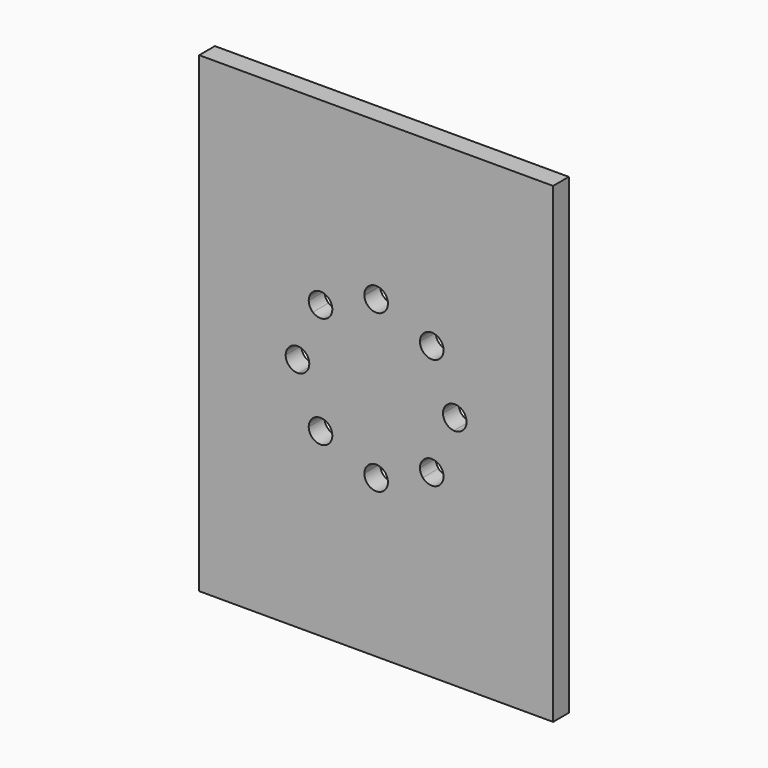
from build123d import *

# Parameters (mm, degrees)
F1_DEPTH = 5
F3_DEPTH = 5
F4_R     = 30
F5_DEPTH = 5
F6_DEPTH = 10


# Not quite as in the source:
# - a feature names something its author has since deleted; it is built from what else it names


with BuildPart() as f1:
    # F0 (on Front) → F1 (new body)
    with BuildSketch(Plane.XZ):
        Polygon((45, 60), (-45, 60), (-45, 0), (-45, -60), (0, -60), (45, -60), align=None)
    extrude(amount=F1_DEPTH)


with BuildPart() as f3:
    # F2 (on face) → F3 (new body)
    with BuildSketch(Plane(origin=(0, 0, 0), x_dir=(-1, 0, 0), z_dir=(0, 1, 0))):
        with BuildLine():
            Line((-40, -45), (-18, -55))
            Line((-18, -55), (18, -55))
            Line((18, -55), (18, -45))
            ThreePointArc((18, -45), (23.4818815859, -37.7525512861), (32.1421356237, -35))
            Line((32.1421356237, -35), (40, -35))
            Line((40, -35), (40, 35))
            Line((40, 35), (33, 35))
            ThreePointArc((33, 35), (22.3933982822, 39.3933982822), (18, 50))
            Line((18, 50), (18, 55))
            Line((18, 55), (-25, 55))
            ThreePointArc((-25, 55), (-35.6066017178, 50.6066017178), (-40, 40))
            Line((-40, 40), (-40, -45))
        make_face()
    extrude(amount=F3_DEPTH)

    # F4 (on face) → F5 (cut)
    with BuildSketch(Plane(origin=(0, 5, 0), x_dir=(-1, 0, 0), z_dir=(0, 1, 0))):
        Circle(F4_R)
        with BuildLine():
            ThreePointArc((16.1001741522, 11.8652598905), (18.4781684496, 7.6522735674), (19.775, 2.9915506013))
            ThreePointArc((19.775, 2.9915506013), (22.0402205763, 2.1994317448), (23, 0))
            ThreePointArc((23, 0), (22.0402205763, -2.1994317448), (19.775, -2.9915506013))
            ThreePointArc((19.775, -2.9915506013), (18.4781684496, -7.6522735674), (16.1001741522, -11.8652598905))
            ThreePointArc((16.1001741522, -11.8652598905), (16.8707805694, -12.8885427857), (17.144270925, -14.14))
            ThreePointArc((17.144270925, -14.14), (15.187715229, -16.9526898131), (11.870121602, -16.0965901095))
            ThreePointArc((11.870121602, -16.0965901095), (7.6550636836, -18.4770127456), (2.9915506013, -19.775))
            ThreePointArc((2.9915506013, -19.775), (2.9978869061, -19.8874207031), (3, -20))
            ThreePointArc((3, -20), (-0.1125792969, -22.9978869061), (-2.9915506013, -19.775))
            ThreePointArc((-2.9915506013, -19.775), (-7.6550636836, -18.4770127456), (-11.870121602, -16.0965901095))
            ThreePointArc((-11.870121602, -16.0965901095), (-16.2659115638, -16.261), (-16.1001741522, -11.8652598905))
            ThreePointArc((-16.1001741522, -11.8652598905), (-18.4781684496, -7.6522735674), (-19.775, -2.9915506013))
            ThreePointArc((-19.775, -2.9915506013), (-23, 0), (-19.775, 2.9915506013))
            ThreePointArc((-19.775, 2.9915506013), (-18.4781684496, 7.6522735674), (-16.1001741522, 11.8652598905))
            ThreePointArc((-16.1001741522, 11.8652598905), (-16.2659115638, 16.261), (-11.870121602, 16.0965901095))
            ThreePointArc((-11.870121602, 16.0965901095), (-7.6550636836, 18.4770127456), (-2.9915506013, 19.775))
            ThreePointArc((-2.9915506013, 19.775), (-0.1125792969, 22.9978869061), (3, 20))
            ThreePointArc((3, 20), (2.9978869061, 19.8874207031), (2.9915506013, 19.775))
            ThreePointArc((2.9915506013, 19.775), (7.6550636836, 18.4770127456), (11.870121602, 16.0965901095))
            ThreePointArc((11.870121602, 16.0965901095), (15.187715229, 16.9526898131), (17.144270925, 14.14))
            ThreePointArc((17.144270925, 14.14), (16.8707805694, 12.8885427857), (16.1001741522, 11.8652598905))
        make_face(mode=Mode.SUBTRACT)
        with BuildLine():
            ThreePointArc((19.775, -2.9915506013), (17, 0), (19.775, 2.9915506013))
            ThreePointArc((19.775, 2.9915506013), (18.4781684496, 7.6522735674), (16.1001741522, 11.8652598905))
            ThreePointArc((16.1001741522, 11.8652598905), (12.0226302863, 12.019), (11.870121602, 16.0965901095))
            ThreePointArc((11.870121602, 16.0965901095), (7.6550636836, 18.4770127456), (2.9915506013, 19.775))
            ThreePointArc((2.9915506013, 19.775), (0, 17), (-2.9915506013, 19.775))
            ThreePointArc((-2.9915506013, 19.775), (-7.6550636836, 18.4770127456), (-11.870121602, 16.0965901095))
            ThreePointArc((-11.870121602, 16.0965901095), (-11.3315811119, 15.183444304), (-11.144270925, 14.14))
            ThreePointArc((-11.144270925, 14.14), (-12.8928137107, 11.4134903556), (-16.1001741522, 11.8652598905))
            ThreePointArc((-16.1001741522, 11.8652598905), (-18.4781684496, 7.6522735674), (-19.775, 2.9915506013))
            ThreePointArc((-19.775, 2.9915506013), (-17.8005682552, 2.0402205763), (-17, 0))
            ThreePointArc((-17, 0), (-17.8005682552, -2.0402205763), (-19.775, -2.9915506013))
            ThreePointArc((-19.775, -2.9915506013), (-18.4781684496, -7.6522735674), (-16.1001741522, -11.8652598905))
            ThreePointArc((-16.1001741522, -11.8652598905), (-12.8928137107, -11.4134903556), (-11.144270925, -14.14))
            ThreePointArc((-11.144270925, -14.14), (-11.3315811119, -15.183444304), (-11.870121602, -16.0965901095))
            ThreePointArc((-11.870121602, -16.0965901095), (-7.6550636836, -18.4770127456), (-2.9915506013, -19.775))
            ThreePointArc((-2.9915506013, -19.775), (0, -17), (2.9915506013, -19.775))
            ThreePointArc((2.9915506013, -19.775), (7.6550636836, -18.4770127456), (11.870121602, -16.0965901095))
            ThreePointArc((11.870121602, -16.0965901095), (12.0226302863, -12.019), (16.1001741522, -11.8652598905))
            ThreePointArc((16.1001741522, -11.8652598905), (18.4781684496, -7.6522735674), (19.775, -2.9915506013))
        make_face()
    extrude(amount=-F5_DEPTH, mode=Mode.SUBTRACT)


with BuildPart() as f6_tool:
    # F6 (cut): faces of the model
    f6_faces = [f3.part.faces().sort_by_distance(p)[0] for p in [
        (14.144270925, 5, -14.14),
        (20, 5, 0),
        (0, 5, 20),
        (14.144270925, 5, 14.14),
        (-14.144270925, 5, 14.14),
        (-20, 5, 0),
        (-14.144270925, 5, -14.14),
        (0, 5, -20),
    ]]
    extrude(f6_faces, amount=-F6_DEPTH)


with BuildPart() as f1_1:
    add(f1.part)

    # F6: cut by f6_tool
    add(f6_tool.part, mode=Mode.SUBTRACT)


with BuildPart() as f3_1:
    add(f3.part)

    # F6: cut by f6_tool
    add(f6_tool.part, mode=Mode.SUBTRACT)


solid = Compound([f1_1.part, f3_1.part])
